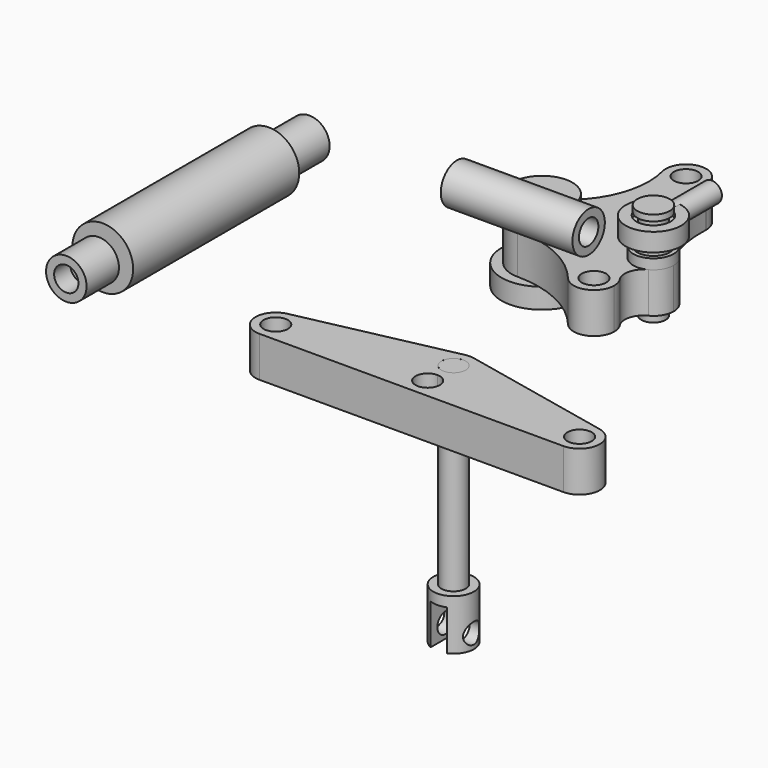
from build123d import *

# Parameters (mm, degrees)
F0_R           = 6
F0_R_2         = 10
F1_DEPTH       = 20
F2_R           = 20
F3_DEPTH       = 10
F4_R           = 10
F5_DEPTH       = 25
F6_R           = 15
F7_DEPTH       = 5
F8_R           = 10
F9_DEPTH       = 5
F10_R          = 8
F11_DEPTH      = 3
F12_R          = 6
F13_DEPTH      = 12
F14_R          = 8
F15_DEPTH      = 3
F16_R          = 6
F17_DEPTH      = 25
F23_R          = 5
F24_DEPTH      = 25
F25_R          = 15
F26_DEPTH      = 100
F27_T          = -2.5
F29_R          = 12.5
F30_DEPTH      = 5
F31_R          = 4
F32_DEPTH      = 100
F33_R          = 15
F33_R_2        = 4
F34_DEPTH      = 2.5
F35_R          = 10
F36_DEPTH      = 20
F38_R          = 6
F39_DEPTH      = 20
F40_R          = 6
F41_DEPTH      = 75
F41_DEPTH_BACK = 20
F42_R          = 10
F43_DEPTH      = 25
F44_W          = 8
F44_H          = 28.0783114423
F45_DEPTH      = 20
F46_R          = 5
F47_DEPTH      = 81.001
F47_DEPTH_BACK = 204.8705715287
F48_R          = 6
F49_DEPTH      = 10
F37_R          = 10
F37_R_2        = 6
F50_DEPTH      = 25
F51_R          = 10
F51_R_2        = 6
F52_DEPTH      = 65


with BuildPart() as f1:
    # F0 (on Top) → F1 (new body)
    with BuildSketch(Plane.XY):
        with BuildLine():
            ThreePointArc((32.2183943562, 60.5719530293), (32.2280800548, 60.8259046296), (32.2313093162, 61.0800203511))
            ThreePointArc((32.2313093162, 61.0800203511), (20.9990439055, 71.0038060177), (12.5350049246, 58.6342727871))
            ThreePointArc((12.5350049246, 58.6342727871), (23.2109978007, 51.1281255328), (32.2183943562, 60.5719530293))
        make_face()
        with Locations((22.2313093162, 61.0800203511)):
            Circle(F0_R, mode=Mode.SUBTRACT)
        with BuildLine():
            ThreePointArc((32.2183943562, 60.5719530293), (23.2109978007, 51.1281255328), (12.5350049246, 58.6342727871))
            ThreePointArc((12.5350049246, 58.6342727871), (10.4025055394, 32.5150172616), (-7.2399984812, 13.1370629135))
            ThreePointArc((-7.2399984812, 13.1370629135), (7.6288931957, 12.9151069918), (15, 0))
            ThreePointArc((15, 0), (10.6066017178, -10.6066017178), (0, -15))
            ThreePointArc((0, -15), (22.0679234012, -19.9499544407), (39.9073868501, -33.8513513514))
            ThreePointArc((39.9073868501, -33.8513513514), (41.731420698, -19.4259503853), (56.0291431418, -22.0706479914))
            ThreePointArc((56.0291431418, -22.0706479914), (54.8697797501, -14.7023131729), (59.5579853088, -8.9008297324))
            ThreePointArc((59.5579853088, -8.9008297324), (45.0047857915, 0.3093427334), (60.0996798249, 8.6019338339))
            ThreePointArc((60.0996798249, 8.6019338339), (38.9221522488, 30.7044424185), (32.2183943562, 60.5719530293))
        make_face()
        with BuildLine():
            ThreePointArc((15, 0), (7.6288931957, 12.9151069918), (-7.2399984812, 13.1370629135))
            ThreePointArc((-7.2399984812, 13.1370629135), (-14.5268018452, -3.737917622), (0, -15))
            ThreePointArc((0, -15), (10.6066017178, -10.6066017178), (15, 0))
        make_face()
        Circle(F0_R_2, mode=Mode.SUBTRACT)
        with BuildLine():
            ThreePointArc((65, 0), (63.688981478, 4.9499091785), (60.0996798249, 8.6019338339))
            ThreePointArc((60.0996798249, 8.6019338339), (45.0047857915, 0.3093427334), (59.5579853088, -8.9008297324))
            ThreePointArc((59.5579853088, -8.9008297324), (63.531701269, -5.2163275833), (65, 0))
        make_face()
        with Locations((55, 0)):
            Circle(F0_R, mode=Mode.SUBTRACT)
        with BuildLine():
            ThreePointArc((56.0291431418, -22.0706479914), (41.731420698, -19.4259503853), (39.9073868501, -33.8513513514))
            ThreePointArc((39.9073868501, -33.8513513514), (51.0048150906, -36.9138223794), (57.6313972081, -27.5))
            ThreePointArc((57.6313972081, -27.5), (57.2224727301, -24.6695812445), (56.0291431418, -22.0706479914))
        make_face()
        with Locations((47.6313972081, -27.5)):
            Circle(F0_R, mode=Mode.SUBTRACT)
    extrude(amount=F1_DEPTH)


with BuildPart() as f3:
    # F2 (on face) → F3 (new body)
    with BuildSketch(Plane(origin=(0, 0, 0), x_dir=(1, 0, 0), z_dir=(0, 0, -1))):
        Circle(F2_R)
    extrude(amount=F3_DEPTH)

    # F4 (on face) → F5 (join)
    with BuildSketch(Plane.XY):
        Circle(F4_R)
    extrude(amount=F5_DEPTH)

    # F6 (on face) → F7 (join)
    with BuildSketch(Plane.XY.offset(25)):
        Circle(F6_R)
    extrude(amount=F7_DEPTH)


with BuildPart() as f9:
    # F8 (on face) → F9 (new body)
    with BuildSketch(Plane.XY.offset(20)):
        with Locations((55, 0)):
            Circle(F8_R)
    extrude(amount=F9_DEPTH)

    # F10 (on face) → F11 (join)
    with BuildSketch(Plane.XY.offset(25)):
        with Locations((55, 0)):
            Circle(F10_R)
    extrude(amount=F11_DEPTH)

    # F12 (on face) → F13 (join)
    with BuildSketch(Plane.XY.offset(28)):
        with Locations((55, 0)):
            Circle(F12_R)
    extrude(amount=F13_DEPTH)

    # F14 (on face) → F15 (join)
    with BuildSketch(Plane.XY.offset(40)):
        with Locations((55, 0)):
            Circle(F14_R)
    extrude(amount=F15_DEPTH)

    # F16 (on face) → F17 (join)
    with BuildSketch(Plane(origin=(0, 0, 20), x_dir=(1, 0, 0), z_dir=(0, 0, -1))):
        with Locations((55, 0)):
            Circle(F16_R)
    extrude(amount=F17_DEPTH)


with BuildPart() as f19:
    # F18 (on Front) → F19 (revolve)
    with BuildSketch(Plane.XZ):
        with BuildLine():
            Line((64.4786655903, 35), (61, 35))
            Line((61, 35), (61, 33))
            Line((61, 33), (64.4786655903, 33))
            ThreePointArc((64.4786655903, 33), (64.5312696621, 34), (64.4786655903, 35))
        make_face()
    revolve(axis=Axis((55, 0, 34), (0, 0, -1)))


with BuildPart() as f21:
    # F20 (on Front) → F21 (revolve)
    with BuildSketch(Plane.XZ):
        with BuildLine():
            Line((68.7309754244, 38.5), (63.4020891076, 38.5))
            ThreePointArc((63.4020891076, 38.5), (64.5312696621, 34), (63.4020891076, 29.5))
            Line((63.4020891076, 29.5), (68.7309754244, 29.5))
            Line((68.7309754244, 29.5), (68.7309754244, 38.5))
        make_face()
    revolve(axis=Axis((55, 0, 33.1719050929), (0, 0, -1)))

    # F23 (on offset) → F24 (join)
    with BuildSketch(Plane.XZ.offset(-11)):
        with Locations((55, 34)):
            Circle(F23_R)
    extrude(amount=-F24_DEPTH)


with BuildPart() as f26:
    # F25 (on Front) → F26 (new body)
    with BuildSketch(Plane.XZ):
        with Locations((-134.871967846, 0)):
            Circle(F25_R)
    extrude(amount=F26_DEPTH)

    # F27
    f27_openings = [f26.faces().sort_by_distance(p)[0] for p in [
        (-134.871968, -100, 0),
    ]]
    offset(amount=F27_T, openings=f27_openings)

    # F33 (on face) → F34 (join)
    with BuildSketch(Plane.XZ.offset(100)):
        with Locations((-134.871967846, 0)):
            Circle(F33_R)
        with Locations((-134.871967846, 0)):
            Circle(F33_R_2, mode=Mode.SUBTRACT)
    extrude(amount=F34_DEPTH)

    # F37 (on face) → F50 (join)
    with BuildSketch(Plane(origin=(0, 0, 0), x_dir=(-1, 0, 0), z_dir=(0, 1, 0))):
        with Locations((134.871967846, 0)):
            Circle(F37_R)
        with Locations((134.871967846, 0)):
            Circle(F37_R_2, mode=Mode.SUBTRACT)
    extrude(amount=F50_DEPTH)


with BuildPart() as f30:
    # F29 (on offset) → F30 (new body)
    with BuildSketch(Plane.XZ):
        with Locations((-134.871967846, 0)):
            Circle(F29_R)
    extrude(amount=F30_DEPTH)

    # F31 (on face) → F32 (join)
    with BuildSketch(Plane.XZ.offset(5)):
        with Locations((-134.871967846, 0)):
            Circle(F31_R)
    extrude(amount=F32_DEPTH)

    # F35 (on face) → F36 (join)
    with BuildSketch(Plane.XZ.offset(105)):
        with Locations((-134.871967846, 0)):
            Circle(F35_R)
    extrude(amount=F36_DEPTH)

    # F48 (on face) → F49 (cut)
    with BuildSketch(Plane.XZ.offset(125)):
        with Locations((-134.871967846, 0)):
            Circle(F48_R)
    extrude(amount=-F49_DEPTH, mode=Mode.SUBTRACT)


with BuildPart() as f39:
    # F38 (on Top) → F39 (new body)
    with BuildSketch(Plane.XY):
        with BuildLine():
            ThreePointArc((56.9976036827, -126.3386778119), (54.1598813303, -127.8255107966), (50.9976036562, -128.3386778119))
            ThreePointArc((50.9976036562, -128.3386778119), (47.83532601, -127.8255107882), (44.9976036827, -126.3386778119))
            ThreePointArc((44.9976036827, -126.3386778119), (41.5107707022, -137.500955472), (50.9976036827, -144.3386778119))
            ThreePointArc((50.9976036827, -144.3386778119), (58.0686714946, -141.4097456237), (60.9976036827, -134.3386778119))
            ThreePointArc((60.9976036827, -134.3386778119), (59.9418755927, -129.8665418569), (56.9976036827, -126.3386778119))
        make_face()
        with BuildLine():
            ThreePointArc((50.9976036562, -128.3386778119), (55.2402443605, -130.0960371154), (56.9976036827, -134.3386778119))
            ThreePointArc((56.9976036827, -134.3386778119), (46.7549630049, -138.5813185083), (50.9976036562, -128.3386778119))
        make_face(mode=Mode.SUBTRACT)
        with BuildLine():
            ThreePointArc((48.911218965, -108.5587494476), (41.2313931786, -116.1889958843), (44.9976036827, -126.3386778119))
            ThreePointArc((44.9976036827, -126.3386778119), (47.8353260225, -124.8518448314), (50.9976036827, -124.3386778119))
            ThreePointArc((50.9976036827, -124.3386778119), (54.1598813429, -124.8518448314), (56.9976036827, -126.3386778119))
            ThreePointArc((56.9976036827, -126.3386778119), (59.9418755927, -122.8108137669), (60.9976036827, -118.3386778119))
            ThreePointArc((60.9976036827, -118.3386778119), (58.7714009266, -112.0483617299), (53.0839884004, -108.5587494476))
            ThreePointArc((53.0839884004, -108.5587494476), (50.9976036827, -108.3386778119), (48.911218965, -108.5587494476))
        make_face()
        with BuildLine():
            ThreePointArc((56.9976036827, -118.3386778119), (55.2402443698, -122.581318499), (50.9976036827, -124.3386778119))
            ThreePointArc((50.9976036827, -124.3386778119), (46.7549629956, -114.0960371248), (56.9976036827, -118.3386778119))
        make_face(mode=Mode.SUBTRACT)
        with BuildLine():
            ThreePointArc((50.9976036827, -144.3386778119), (41.5107707022, -137.500955472), (44.9976036827, -126.3386778119))
            ThreePointArc((44.9976036827, -126.3386778119), (41.2313931786, -116.1889958843), (48.911218965, -108.5587494476))
            Line((48.911218965, -108.5587494476), (-26.088781035, -124.5587494476))
            ThreePointArc((-26.088781035, -124.5587494476), (-17.7120802353, -126.564880568), (-14.0023963173, -134.3386778119))
            ThreePointArc((-14.0023963173, -134.3386778119), (-16.9313285054, -141.4097456237), (-24.0023963173, -144.3386778119))
            Line((-24.0023963173, -144.3386778119), (50.9976036827, -144.3386778119))
        make_face()
        with BuildLine():
            ThreePointArc((60.9976036827, -118.3386778119), (59.9418755927, -122.8108137669), (56.9976036827, -126.3386778119))
            ThreePointArc((56.9976036827, -126.3386778119), (59.9418755927, -129.8665418569), (60.9976036827, -134.3386778119))
            ThreePointArc((60.9976036827, -134.3386778119), (58.0686714946, -141.4097456237), (50.9976036827, -144.3386778119))
            Line((50.9976036827, -144.3386778119), (125.9976036827, -144.3386778119))
            ThreePointArc((125.9976036827, -144.3386778119), (116.0527737786, -133.2896982226), (128.0839884004, -124.5587494476))
            Line((128.0839884004, -124.5587494476), (53.0839884004, -108.5587494476))
            ThreePointArc((53.0839884004, -108.5587494476), (58.7714009266, -112.0483617299), (60.9976036827, -118.3386778119))
        make_face()
        with BuildLine():
            ThreePointArc((-26.088781035, -124.5587494476), (-33.9472262214, -135.3876574012), (-24.0023963173, -144.3386778119))
            ThreePointArc((-24.0023963173, -144.3386778119), (-16.9313285054, -141.4097456237), (-14.0023963173, -134.3386778119))
            ThreePointArc((-14.0023963173, -134.3386778119), (-17.7120802353, -126.564880568), (-26.088781035, -124.5587494476))
        make_face()
        with Locations((-24.0023963173, -134.3386778119)):
            Circle(F38_R, mode=Mode.SUBTRACT)
        with BuildLine():
            ThreePointArc((128.0839884004, -124.5587494476), (116.0527737786, -133.2896982226), (125.9976036827, -144.3386778119))
            ThreePointArc((125.9976036827, -144.3386778119), (133.0686714946, -141.4097456237), (135.9976036827, -134.3386778119))
            ThreePointArc((135.9976036827, -134.3386778119), (133.7714009266, -128.0483617299), (128.0839884004, -124.5587494476))
        make_face()
        with Locations((125.9976036827, -134.3386778119)):
            Circle(F38_R, mode=Mode.SUBTRACT)
        with BuildLine():
            ThreePointArc((44.9976036827, -126.3386778119), (47.83532601, -127.8255107882), (50.9976036562, -128.3386778119))
            ThreePointArc((50.9976036562, -128.3386778119), (54.1598813303, -127.8255107966), (56.9976036827, -126.3386778119))
            ThreePointArc((56.9976036827, -126.3386778119), (54.1598813429, -124.8518448314), (50.9976036827, -124.3386778119))
            ThreePointArc((50.9976036827, -124.3386778119), (47.8353260225, -124.8518448314), (44.9976036827, -126.3386778119))
        make_face()
    extrude(amount=F39_DEPTH)


with BuildPart() as f41:
    # F40 (on face) → F41 (new body, two sides)
    with BuildSketch(Plane(origin=(0, 0, 0), x_dir=(1, 0, 0), z_dir=(0, 0, -1))) as f41_sk:
        with Locations((50.9976036827, 118.3386778119)):
            Circle(F40_R)
    extrude(amount=F41_DEPTH)
    extrude(f41_sk.sketch, amount=-F41_DEPTH_BACK)

    # F42 (on face) → F43 (join)
    with BuildSketch(Plane(origin=(0, 0, -75), x_dir=(1, 0, 0), z_dir=(0, 0, -1))):
        with Locations((50.9976036827, 118.3386778119)):
            Circle(F42_R)
    extrude(amount=F43_DEPTH)

    # F44 (on face) → F45 (cut)
    with BuildSketch(Plane(origin=(0, 0, -100), x_dir=(1, 0, 0), z_dir=(0, 0, -1))):
        with Locations((50.9976036827, 118.3386778119)):
            Rectangle(F44_W, F44_H)
    extrude(amount=-F45_DEPTH, mode=Mode.SUBTRACT)

    # F46 (on face) → F47 (cut, two sides)
    with BuildSketch(Plane(origin=(54.9976036827, 0, 0), x_dir=(0, -1, 0), z_dir=(-1, 0, 0))) as f47_sk:
        with Locations((118.3386778119, -93)):
            Circle(F46_R)
    extrude(amount=-F47_DEPTH, mode=Mode.SUBTRACT)
    extrude(f47_sk.sketch, amount=F47_DEPTH_BACK, mode=Mode.SUBTRACT)


with BuildPart() as f52:
    # F51 (on Right) → F52 (new body)
    with BuildSketch(Plane.YZ):
        with Locations((-52.5045208633, 55.8896288276)):
            Circle(F51_R)
        with Locations((-52.5045208633, 55.8896288276)):
            Circle(F51_R_2, mode=Mode.SUBTRACT)
    extrude(amount=F52_DEPTH)


solid = Compound([f1.part, f3.part, f9.part, f19.part, f21.part, f26.part, f30.part, f39.part, f41.part, f52.part])
